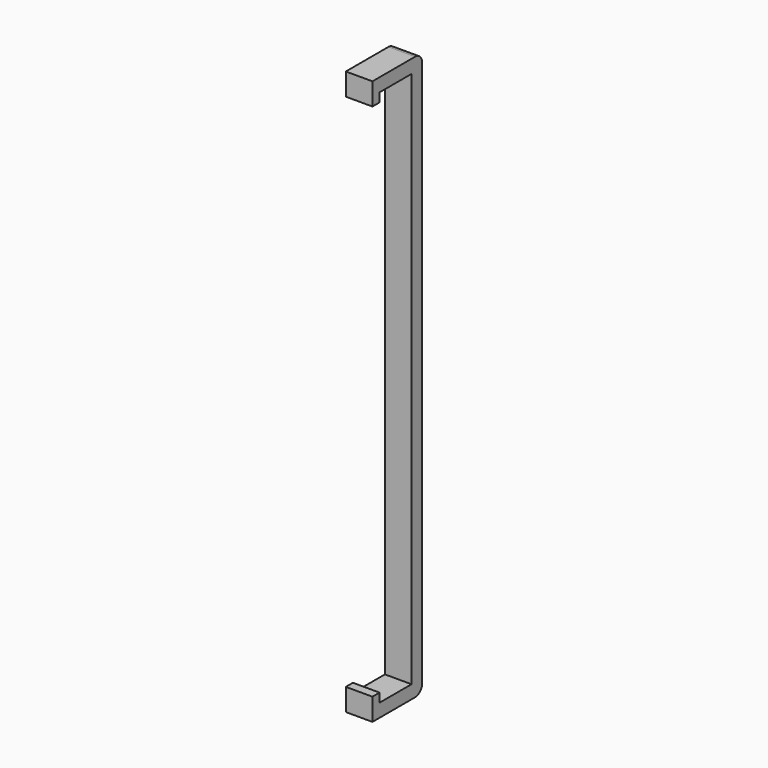
from build123d import *

# Parameters (mm, degrees)
F1_DEPTH = 7.62
F2_R     = 2.54


# Not quite as in the source:
# - a feature names something its author has since deleted; it is built from what else it names


with BuildPart() as f1:
    # F0 (on Right) → F1 (new body)
    with BuildSketch(Plane.YZ):
        Polygon((-39.391245693, -75.0930126251), (-21.611245693, -75.0930126251), (-21.611245693, 86.1969873749), (-36.851245693, 86.1969873749), (-39.391245693, 86.1969873749), (-39.391245693, 79.8469873749), (-36.851245693, 79.8469873749), (-36.851245693, 82.3869873749), (-25.421245693, 82.3869873749), (-25.421245693, -71.2830126251), (-36.851245693, -71.2830126251), (-36.851245693, -68.7430126251), (-39.391245693, -68.7430126251), align=None)
    extrude(amount=F1_DEPTH)

    # F2
    f2_edges = [f1.edges().sort_by_distance(p)[0] for p in [
        (3.81, -21.611246, -75.093013),
        (3.81, -21.611246, 86.196987),
    ]]
    fillet(f2_edges, radius=F2_R)


solid = f1.part
